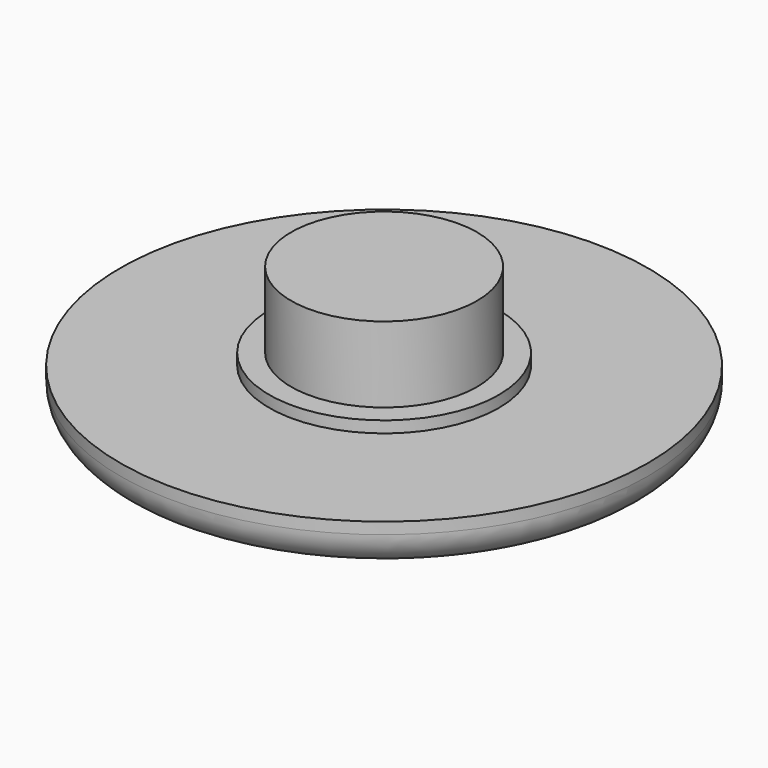
from build123d import *

# Parameters (mm, degrees)
F0_R     = 11.5
F1_DEPTH = 2
F2_R     = 5
F3_DEPTH = 0.5
F4_R     = 4.05
F5_DEPTH = 3.3
F6_R     = 10
F7_DEPTH = 1
F9_R     = 1.49999


# Not quite as in the source:
# - a fillet or chamfer that OpenCascade refuses, or shapes differently, is made with other operations: its cross-section is extruded or revolved along the edge and cut away or added
# - a fillet or chamfer is up to 0.001 mm smaller than in the source, because OpenCascade refuses the exact size


with BuildPart() as f1:
    # F0 (on Top) → F1 (new body)
    with BuildSketch(Plane.XY):
        Circle(F0_R)
    extrude(amount=F1_DEPTH)

    # F2 (on face) → F3 (join)
    with BuildSketch(Plane.XY.offset(2)):
        Circle(F2_R)
    extrude(amount=F3_DEPTH)

    # F4 (on face) → F5 (join)
    with BuildSketch(Plane.XY.offset(2.5)):
        Circle(F4_R)
    extrude(amount=F5_DEPTH)

    # F6 (on face) → F7 (cut)
    with BuildSketch(Plane(origin=(0, 0, 0), x_dir=(1, 0, 0), z_dir=(0, 0, -1))):
        Circle(F6_R)
    extrude(amount=-F7_DEPTH, mode=Mode.SUBTRACT)

    # F8: fillet of radius 32 on 1 edges, made by hand

    # F8_s1 → F8_t2 (revolve)
    with BuildSketch(Plane.XZ):
        with BuildLine():
            ThreePointArc((10, 0), (6.0627460668, 0.7490157328), (2.0627460668, 1))
            Line((2.0627460668, 1), (10, 1))
            Line((10, 1), (10, 0))
        make_face()
    revolve(axis=Axis((0, 0, 1), (0, 0, -1)))

    # F9 (radius 1.5 in the source; OpenCascade refuses exactly that, so slightly less here)
    f9_edges = [f1.edges().sort_by_distance(p)[0] for p in [
        (-11.5, 0, 0),
    ]]
    fillet(f9_edges, radius=F9_R)


solid = f1.part
